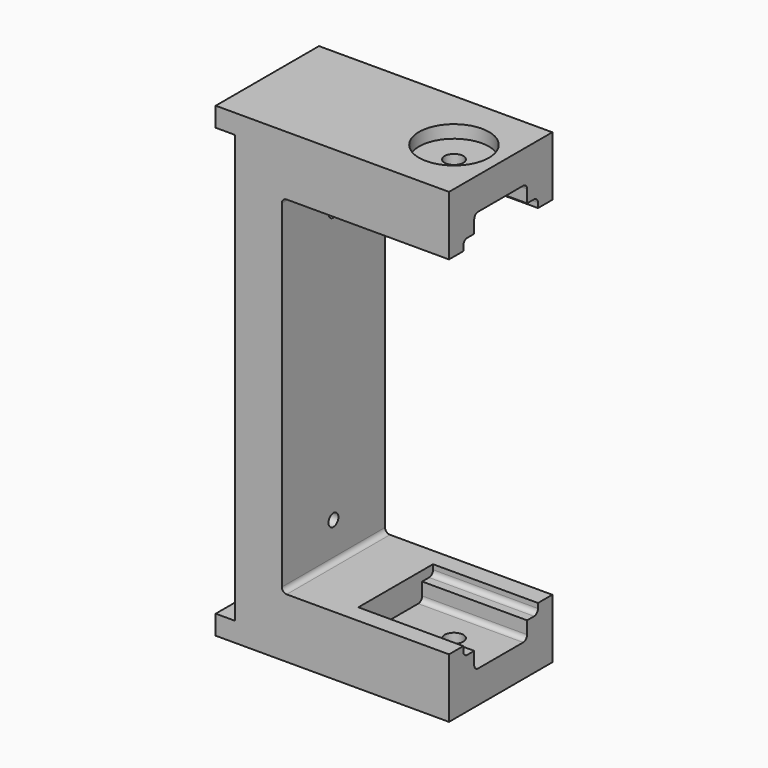
from build123d import *

# Parameters (mm, degrees)
F0_W      = 76.2
F0_H      = 42.164
F1_DEPTH  = 152.4
F3_DEPTH  = 42.165
F5_DEPTH  = 34.29
F7_R      = 11.43
F8_DEPTH  = 4.191
F9_R      = 3.048
F10_DEPTH = 6.35
F12_DEPTH = 6.35
F14_D     = 4.0386


# Not quite as in the source:
# - a pattern or mirror of a feature is missing from the dataset's text; its kind, count and spacing are read off the source's solid


with BuildPart() as f1:
    # F0 (on Top) → F1 (new body)
    with BuildSketch(Plane.XY):
        with Locations((38.1, 21.082)):
            Rectangle(F0_W, F0_H)
    extrude(amount=F1_DEPTH)

    # F2 (on face) → F3 (cut, through all)
    with BuildSketch(Plane.XZ):
        with BuildLine():
            Line((23.1775, 19.431), (76.2, 19.431))
            Line((76.2, 19.431), (76.2, 132.969))
            Line((76.2, 132.969), (23.1775, 132.969))
            ThreePointArc((23.1775, 132.969), (22.0549679849, 132.5040320151), (21.59, 131.3815))
            Line((21.59, 131.3815), (21.59, 21.0185))
            ThreePointArc((21.59, 21.0185), (22.0549679849, 19.8959679849), (23.1775, 19.431))
        make_face()
    extrude(amount=-F3_DEPTH, mode=Mode.SUBTRACT)

    # F4 (on face) → F5 (cut)
    with BuildSketch(Plane.YZ.offset(76.2)):
        with BuildLine():
            Line((36.322, 17.8435), (36.322, 19.431))
            Line((36.322, 19.431), (5.842, 19.431))
            Line((5.842, 19.431), (5.842, 17.8435))
            ThreePointArc((5.842, 17.8435), (6.3069679849, 16.7209679849), (7.4295, 16.256))
            Line((7.4295, 16.256), (10.287, 16.256))
            Line((10.287, 16.256), (10.287, 12.1285))
            ThreePointArc((10.287, 12.1285), (10.7519679849, 11.0059679849), (11.8745, 10.541))
            Line((11.8745, 10.541), (30.2895, 10.541))
            ThreePointArc((30.2895, 10.541), (31.4120320151, 11.0059679849), (31.877, 12.1285))
            Line((31.877, 12.1285), (31.877, 16.256))
            Line((31.877, 16.256), (34.7345, 16.256))
            ThreePointArc((34.7345, 16.256), (35.8570320151, 16.7209679849), (36.322, 17.8435))
        make_face()
    f5 = extrude(amount=-F5_DEPTH, mode=Mode.SUBTRACT)

    # F5_copies: F5 across plane
    add(f5.mirror(Plane.XY.offset(76.2)), mode=Mode.SUBTRACT)

    # F7 (on face) → F8 (cut)
    with BuildSketch(Plane(origin=(0, 0, 0), x_dir=(1, 0, 0), z_dir=(0, 0, -1))):
        with Locations((60.96, -21.082)):
            Circle(F7_R)
    f8 = extrude(amount=-F8_DEPTH, mode=Mode.SUBTRACT)

    # F8_copies: F8 across plane
    add(f8.mirror(Plane.XY.offset(76.2)), mode=Mode.SUBTRACT)

    # F9 (on face) → F10 (cut, through all)
    with BuildSketch(Plane(origin=(0, 0, 4.191), x_dir=(1, 0, 0), z_dir=(0, 0, -1))):
        with Locations((60.96, -21.082)):
            Circle(F9_R)
    f10 = extrude(amount=-F10_DEPTH, mode=Mode.SUBTRACT)

    # F10_copies: F10 across plane
    add(f10.mirror(Plane.XY.offset(76.2)), mode=Mode.SUBTRACT)

    # F11 (on face) → F12 (cut)
    with BuildSketch(Plane(origin=(0, 0, 0), x_dir=(0, -1, 0), z_dir=(-1, 0, 0))):
        with BuildLine():
            Line((-32.639, 6.35), (0, 6.35))
            Line((0, 6.35), (0, 146.05))
            Line((0, 146.05), (-32.639, 146.05))
            ThreePointArc((-32.639, 146.05), (-34.8840640303, 145.1200640303), (-35.814, 142.875))
            Line((-35.814, 142.875), (-35.814, 9.525))
            ThreePointArc((-35.814, 9.525), (-34.8840640303, 7.2799359697), (-32.639, 6.35))
        make_face()
    extrude(amount=-F12_DEPTH, mode=Mode.SUBTRACT)

    # F14 (through all)
    with Locations(Plane(origin=(6.35, 0, 0), x_dir=(0, -1, 0), z_dir=(-1, 0, 0))):
        with Locations((-21.082, 120.65), (-21.082, 31.75)):
            Hole(F14_D / 2)


solid = f1.part
